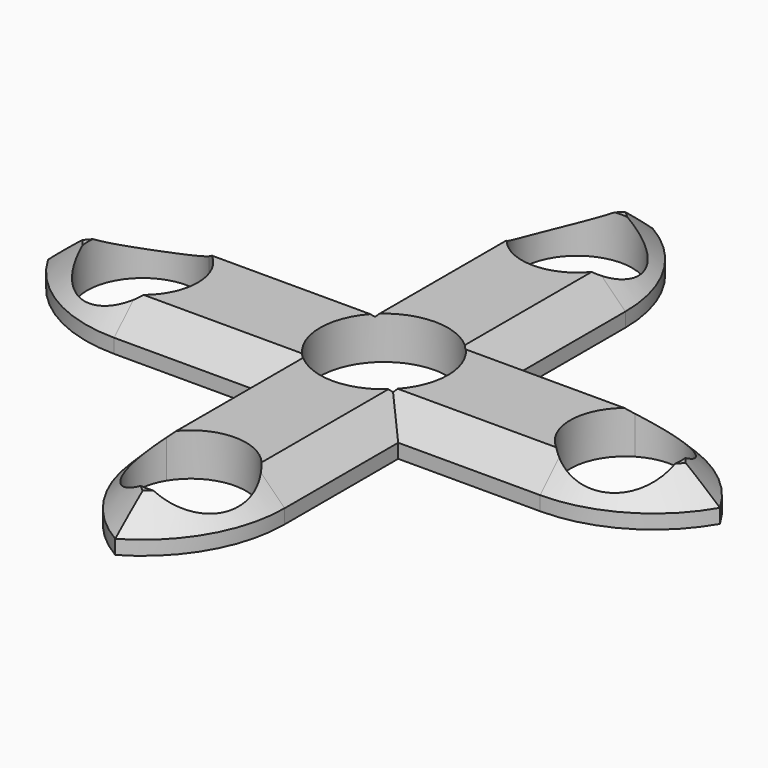
from build123d import *

# Parameters (mm, degrees)
F0_W         = 25.4
F0_H         = 25.4
F0_R         = 11.45
F1_DEPTH     = 7.62
F2_T1_DEPTH  = 25.4
F2_T3_DEPTH  = 25.4
F2_T5_DEPTH  = 25.4
F2_T7_DEPTH  = 25.4
F2_T10_ANGLE = 89.4745768315
F2_T12_ANGLE = 89.4745768315
F2_T14_ANGLE = 89.4745768315
F2_T16_ANGLE = 89.4745768315
F2_T18_ANGLE = 89.4745768315
F2_T20_ANGLE = 89.4745768315
F2_T22_ANGLE = 89.4745768315
F2_T24_ANGLE = 89.4745768315
F2_T29_DEPTH = 38.4641495789
F2_T33_DEPTH = 38.4641495789
F2_T40_DEPTH = 38.4641495789
F2_T44_DEPTH = 38.4641495789
F2_T51_DEPTH = 38.4641495789
F2_T55_DEPTH = 38.4641495789
F2_T62_DEPTH = 38.4641495789
F2_T66_DEPTH = 38.4641495789


# Not quite as in the source:
# - a fillet or chamfer that OpenCascade refuses, or shapes differently, is made with other operations: its cross-section is extruded or revolved along the edge and cut away or added


with BuildPart() as f1:
    # F0 (on Top) → F1 (new body)
    with BuildSketch(Plane.XY):
        Rectangle(F0_W, F0_H)
        Circle(F0_R, mode=Mode.SUBTRACT)
        with BuildLine():
            Line((8.4598493137, -38.1), (12.7, -38.1))
            Line((12.7, -38.1), (12.7, -12.7))
            Line((12.7, -12.7), (-12.7, -12.7))
            Line((-12.7, -12.7), (-12.7, -38.1))
            Line((-12.7, -38.1), (-8.4598493137, -38.1))
            ThreePointArc((-8.4598493137, -38.1), (0, -33.3121), (8.4598493137, -38.1))
        make_face()
        with BuildLine():
            ThreePointArc((0, -60.0970452561), (9.2970452561, -50.8), (12.7, -38.1))
            Line((12.7, -38.1), (8.4598493137, -38.1))
            ThreePointArc((8.4598493137, -38.1), (9.5093742552, -40.5442360341), (9.8679, -43.18))
            ThreePointArc((9.8679, -43.18), (-2.6357639659, -52.6893742552), (-8.4598493137, -38.1))
            Line((-8.4598493137, -38.1), (-12.7, -38.1))
            ThreePointArc((-12.7, -38.1), (-9.2970452561, -50.8), (0, -60.0970452561))
        make_face()
        with BuildLine():
            Line((38.1, -8.4598493137), (38.1, -12.7))
            ThreePointArc((38.1, -12.7), (50.8, -9.2970452561), (60.0970452561, 0))
            ThreePointArc((60.0970452561, 0), (50.8, 9.2970452561), (38.1, 12.7))
            Line((38.1, 12.7), (38.1, 8.4598493137))
            ThreePointArc((38.1, 8.4598493137), (48.0403764468, 8.5879095946), (53.0479, 0))
            ThreePointArc((53.0479, 0), (48.0403764468, -8.5879095946), (38.1, -8.4598493137))
        make_face()
        with BuildLine():
            Line((12.7, 12.7), (12.7, -12.7))
            Line((12.7, -12.7), (38.1, -12.7))
            Line((38.1, -12.7), (38.1, -8.4598493137))
            ThreePointArc((38.1, -8.4598493137), (33.3121, 0), (38.1, 8.4598493137))
            Line((38.1, 8.4598493137), (38.1, 12.7))
            Line((38.1, 12.7), (12.7, 12.7))
        make_face()
        with BuildLine():
            Line((-12.7, 12.7), (12.7, 12.7))
            Line((12.7, 12.7), (12.7, 38.1))
            Line((12.7, 38.1), (8.4598493137, 38.1))
            ThreePointArc((8.4598493137, 38.1), (0, 33.3121), (-8.4598493137, 38.1))
            Line((-8.4598493137, 38.1), (-12.7, 38.1))
            Line((-12.7, 38.1), (-12.7, 12.7))
        make_face()
        with BuildLine():
            Line((8.4598493137, 38.1), (12.7, 38.1))
            ThreePointArc((12.7, 38.1), (9.2970452561, 50.8), (0, 60.0970452561))
            ThreePointArc((0, 60.0970452561), (-9.2970452561, 50.8), (-12.7, 38.1))
            Line((-12.7, 38.1), (-8.4598493137, 38.1))
            ThreePointArc((-8.4598493137, 38.1), (-2.6357639659, 52.6893742552), (9.8679, 43.18))
            ThreePointArc((9.8679, 43.18), (9.5093742552, 40.5442360341), (8.4598493137, 38.1))
        make_face()
        with BuildLine():
            ThreePointArc((-60.0970452561, 0), (-50.8, -9.2970452561), (-38.1, -12.7))
            Line((-38.1, -12.7), (-38.1, -8.4598493137))
            ThreePointArc((-38.1, -8.4598493137), (-53.0479, 0), (-38.1, 8.4598493137))
            Line((-38.1, 8.4598493137), (-38.1, 12.7))
            ThreePointArc((-38.1, 12.7), (-50.8, 9.2970452561), (-60.0970452561, 0))
        make_face()
        with BuildLine():
            Line((-38.1, -12.7), (-12.7, -12.7))
            Line((-12.7, -12.7), (-12.7, 12.7))
            Line((-12.7, 12.7), (-38.1, 12.7))
            Line((-38.1, 12.7), (-38.1, 8.4598493137))
            ThreePointArc((-38.1, 8.4598493137), (-34.5920904054, 4.8603764468), (-33.3121, 0))
            ThreePointArc((-33.3121, 0), (-34.5920904054, -4.8603764468), (-38.1, -8.4598493137))
            Line((-38.1, -8.4598493137), (-38.1, -12.7))
        make_face()
    extrude(amount=F1_DEPTH)

    # F2: chamfer of 5.08 on 8 edges, made by hand

    # F2_s2 → F2_t1 (cut)
    with BuildSketch(Plane.YZ.offset(-38.1)):
        Polygon((-12.7, 2.54), (-7.62, 7.62), (-12.7, 7.62), align=None)
        Polygon((12.7, 2.54), (7.62, 7.62), (12.7, 7.62), align=None)
    extrude(amount=F2_T1_DEPTH, mode=Mode.SUBTRACT)

    # F2_s4 → F2_t3 (cut)
    with BuildSketch(Plane.XZ.offset(12.7)):
        Polygon((-12.7, 2.54), (-7.62, 7.62), (-12.7, 7.62), align=None)
        Polygon((12.7, 2.54), (7.62, 7.62), (12.7, 7.62), align=None)
    extrude(amount=F2_T3_DEPTH, mode=Mode.SUBTRACT)

    # F2_s6 → F2_t5 (cut)
    with BuildSketch(Plane.YZ.offset(12.7)):
        Polygon((-12.7, 2.54), (-7.62, 7.62), (-12.7, 7.62), align=None)
        Polygon((12.7, 2.54), (7.62, 7.62), (12.7, 7.62), align=None)
    extrude(amount=F2_T5_DEPTH, mode=Mode.SUBTRACT)

    # F2_s8 → F2_t7 (cut)
    with BuildSketch(Plane.XZ.offset(-38.1)):
        Polygon((12.7, 2.54), (7.62, 7.62), (12.7, 7.62), align=None)
        Polygon((-12.7, 2.54), (-7.62, 7.62), (-12.7, 7.62), align=None)
    extrude(amount=F2_T7_DEPTH, mode=Mode.SUBTRACT)

    # F2_s9 → F2_t10 (revolve, cut)
    with BuildSketch(Plane.YZ.offset(-38.1)):
        Polygon((12.7, 2.54), (7.62, 7.62), (12.7, 7.62), align=None)
    revolve(axis=Axis((-38.1, -12.7, 7.62), (0, 0, 1)), revolution_arc=F2_T10_ANGLE, mode=Mode.SUBTRACT)

    # F2_s11 → F2_t12 (revolve, cut)
    with BuildSketch(Plane(origin=(13.0483033064, 0.1196610486, 0), x_dir=(0, 0, 1), z_dir=(0.9999579525, 0.0091702357, 0))):
        Polygon((2.54, -63.3819359967), (7.62, -58.3019359967), (7.62, -63.3819359967), align=None)
    revolve(axis=Axis((12.7, 38.1, 7.62), (0, 0, 1)), revolution_arc=F2_T12_ANGLE, mode=Mode.SUBTRACT)

    # F2_s13 → F2_t14 (revolve, cut)
    with BuildSketch(Plane.XZ.offset(-38.1)):
        Polygon((12.7, 2.54), (7.62, 7.62), (12.7, 7.62), align=None)
    revolve(axis=Axis((-12.7, 38.1, 7.62), (0, 0, 1)), revolution_arc=F2_T14_ANGLE, mode=Mode.SUBTRACT)

    # F2_s15 → F2_t16 (revolve, cut)
    with BuildSketch(Plane(origin=(0.1196610486, -13.0483033064, 0), x_dir=(0, 0, 1), z_dir=(0.0091702357, -0.9999579525, 0))):
        Polygon((2.54, -63.3819359967), (7.62, -58.3019359967), (7.62, -63.3819359967), align=None)
    revolve(axis=Axis((38.1, -12.7, 7.62), (0, 0, 1)), revolution_arc=F2_T16_ANGLE, mode=Mode.SUBTRACT)

    # F2_s17 → F2_t18 (revolve, cut)
    with BuildSketch(Plane.YZ.offset(38.1)):
        Polygon((-12.7, 2.54), (-7.62, 7.62), (-12.7, 7.62), align=None)
    revolve(axis=Axis((38.1, 12.7, 7.62), (0, 0, 1)), revolution_arc=F2_T18_ANGLE, mode=Mode.SUBTRACT)

    # F2_s19 → F2_t20 (revolve, cut)
    with BuildSketch(Plane(origin=(-13.0483033064, -0.1196610486, 0), x_dir=(0, 0, 1), z_dir=(-0.9999579525, -0.0091702357, 0))):
        Polygon((2.54, -63.3819359967), (7.62, -58.3019359967), (7.62, -63.3819359967), align=None)
    revolve(axis=Axis((-12.7, -38.1, 7.62), (0, 0, 1)), revolution_arc=F2_T20_ANGLE, mode=Mode.SUBTRACT)

    # F2_s21 → F2_t22 (revolve, cut)
    with BuildSketch(Plane.XZ.offset(38.1)):
        Polygon((-12.7, 2.54), (-7.62, 7.62), (-12.7, 7.62), align=None)
    revolve(axis=Axis((12.7, -38.1, 7.62), (0, 0, 1)), revolution_arc=F2_T22_ANGLE, mode=Mode.SUBTRACT)

    # F2_s23 → F2_t24 (revolve, cut)
    with BuildSketch(Plane(origin=(-0.1196610486, 13.0483033064, 0), x_dir=(0, 0, 1), z_dir=(-0.0091702357, 0.9999579525, 0))):
        Polygon((2.54, -63.3819359967), (7.62, -58.3019359967), (7.62, -63.3819359967), align=None)
    revolve(axis=Axis((-38.1, 12.7, 7.62), (0, 0, 1)), revolution_arc=F2_T24_ANGLE, mode=Mode.SUBTRACT)


with BuildPart() as f2_tool27:
    # F2_s28 → F2_t29 (new body)
    with BuildSketch(Plane.YZ.offset(-38.1)):
        Polygon((-12.7, 2.54), (-7.62, 7.62), (-12.7, 7.62), align=None)
    extrude(amount=F2_T29_DEPTH)

    split(bisect_by=Plane.YZ.offset(-12.7), keep=Keep.TOP)


with BuildPart() as f2_tool31:
    # F2_s32 → F2_t33 (new body)
    with BuildSketch(Plane.XZ.offset(-0.3641495789)):
        Polygon((-12.7, 2.54), (-7.62, 7.62), (-12.7, 7.62), align=None)
    extrude(amount=F2_T33_DEPTH)

    split(bisect_by=Plane.XZ.offset(12.7), keep=Keep.BOTTOM)


with BuildPart() as f2_tool27_1:
    add(f2_tool27.part)

    # F2_t35: intersect F2_tool31
    add(f2_tool31.part, mode=Mode.INTERSECT)


with BuildPart() as f1_1:
    add(f1.part)

    # F2_t25: cut F2_tool27
    add(f2_tool27_1.part, mode=Mode.SUBTRACT)


with BuildPart() as f2_tool38:
    # F2_s39 → F2_t40 (new body)
    with BuildSketch(Plane.XZ.offset(38.1)):
        Polygon((12.7, 2.54), (7.62, 7.62), (12.7, 7.62), align=None)
    extrude(amount=-F2_T40_DEPTH)

    split(bisect_by=Plane.XZ.offset(12.7), keep=Keep.BOTTOM)


with BuildPart() as f2_tool42:
    # F2_s43 → F2_t44 (new body)
    with BuildSketch(Plane.YZ.offset(-0.3641495789)):
        Polygon((-12.7, 2.54), (-7.62, 7.62), (-12.7, 7.62), align=None)
    extrude(amount=F2_T44_DEPTH)

    split(bisect_by=Plane.YZ.offset(12.7), keep=Keep.BOTTOM)


with BuildPart() as f2_tool38_1:
    add(f2_tool38.part)

    # F2_t46: intersect F2_tool42
    add(f2_tool42.part, mode=Mode.INTERSECT)


with BuildPart() as f1_2:
    add(f1_1.part)

    # F2_t36: cut F2_tool38
    add(f2_tool38_1.part, mode=Mode.SUBTRACT)


with BuildPart() as f2_tool49:
    # F2_s50 → F2_t51 (new body)
    with BuildSketch(Plane.YZ.offset(38.1)):
        Polygon((12.7, 2.54), (7.62, 7.62), (12.7, 7.62), align=None)
    extrude(amount=-F2_T51_DEPTH)

    split(bisect_by=Plane.YZ.offset(12.7), keep=Keep.BOTTOM)


with BuildPart() as f2_tool53:
    # F2_s54 → F2_t55 (new body)
    with BuildSketch(Plane.XZ.offset(0.3641495789)):
        Polygon((12.7, 2.54), (7.62, 7.62), (12.7, 7.62), align=None)
    extrude(amount=-F2_T55_DEPTH)

    split(bisect_by=Plane.XZ.offset(-12.7), keep=Keep.TOP)


with BuildPart() as f2_tool49_1:
    add(f2_tool49.part)

    # F2_t57: intersect F2_tool53
    add(f2_tool53.part, mode=Mode.INTERSECT)


with BuildPart() as f1_3:
    add(f1_2.part)

    # F2_t47: cut F2_tool49
    add(f2_tool49_1.part, mode=Mode.SUBTRACT)


with BuildPart() as f2_tool60:
    # F2_s61 → F2_t62 (new body)
    with BuildSketch(Plane.XZ.offset(-38.1)):
        Polygon((-12.7, 2.54), (-7.62, 7.62), (-12.7, 7.62), align=None)
    extrude(amount=F2_T62_DEPTH)

    split(bisect_by=Plane.XZ.offset(-12.7), keep=Keep.TOP)


with BuildPart() as f2_tool64:
    # F2_s65 → F2_t66 (new body)
    with BuildSketch(Plane.YZ.offset(0.3641495789)):
        Polygon((12.7, 2.54), (7.62, 7.62), (12.7, 7.62), align=None)
    extrude(amount=-F2_T66_DEPTH)

    split(bisect_by=Plane.YZ.offset(-12.7), keep=Keep.TOP)


with BuildPart() as f2_tool60_1:
    add(f2_tool60.part)

    # F2_t68: intersect F2_tool64
    add(f2_tool64.part, mode=Mode.INTERSECT)


with BuildPart() as f1_4:
    add(f1_3.part)

    # F2_t58: cut F2_tool60
    add(f2_tool60_1.part, mode=Mode.SUBTRACT)


solid = f1_4.part
